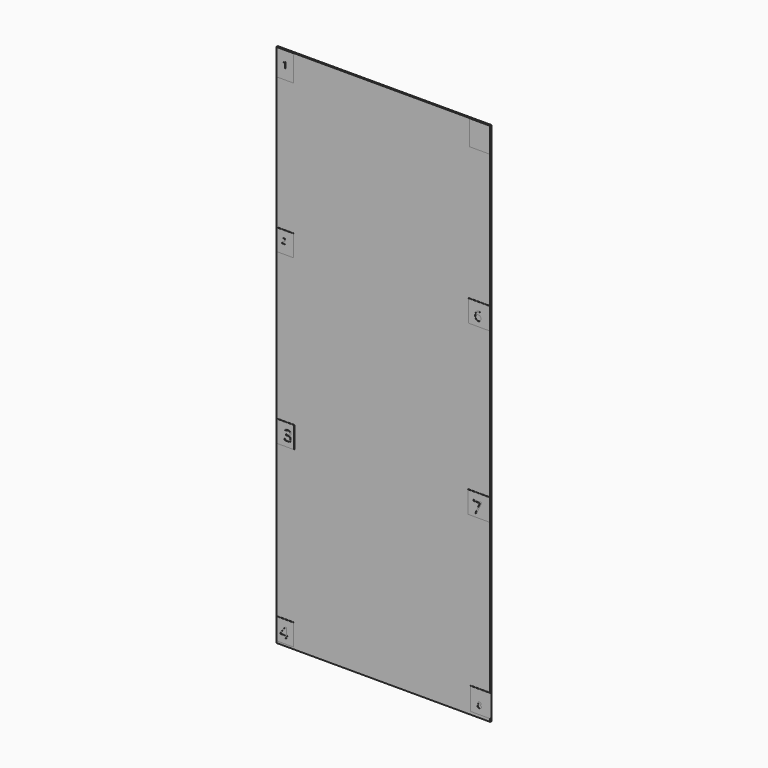
from build123d import *

# Parameters (mm, degrees)
F0_W         = 3500
F0_H         = 8600
F1_DEPTH     = 25
F2_W         = 335
F2_H         = 410
F2_W_2       = 360
F2_H_2       = 360
F2_W_3       = 345
F2_H_3       = 370
F2_W_4       = 350
F2_W_5       = 280
F2_H_4       = 430
F2_W_6       = 290
F2_H_5       = 355
F2_H_6       = 350
F2_TEXT_SIZE = 244.8439598083
F3_DEPTH     = 5


# Not quite as in the source:
# - Text() gives the source's letters only with a copy of the font that has no kerning and outlines rounded to 1/6400 em; it was checked with that copy


with BuildPart() as f1:
    # F0 (on Front) → F1 (new body)
    with BuildSketch(Plane.XZ):
        with Locations((-20.3130850568, 3129.9097295289)):
            Rectangle(F0_W, F0_H)
    extrude(amount=F1_DEPTH)

    # F2 (on face) → F3 (join)
    with BuildSketch(Plane.XZ.offset(25)):
        with Locations((1562.1869149432, 7224.9097295289)):
            Rectangle(F2_W, F2_H)
        with BuildLine():
            add(Edge.make_bspline(
                [(1530.7536032051, 7194.8450300843), (1544.4878190756, 7197.5995246321), (1558.1455212086, 7197.5995246321)],
                knots=[0, 0, 0, 1, 1, 1], degree=2))
            add(Edge.make_bspline(
                [(1558.1455212086, 7197.5995246321), (1585.7669804245, 7197.5995246321), (1601.6053240746, 7183.9035656303)],
                knots=[0, 0, 0, 1, 1, 1], degree=2))
            add(Edge.make_bspline(
                [(1601.6053240746, 7183.9035656303), (1617.4436677247, 7170.2076066285), (1617.4436677247, 7146.4118342847)],
                knots=[0, 0, 0, 1, 1, 1], degree=2))
            add(Edge.make_bspline(
                [(1617.4436677247, 7146.4118342847), (1617.4436677247, 7119.2877143621), (1600.1706914976, 7103.8510678336)],
                knots=[0, 0, 0, 1, 1, 1], degree=2))
            add(Edge.make_bspline(
                [(1600.1706914976, 7103.8510678336), (1582.8977152705, 7088.4144213051), (1552.5217615068, 7088.4144213051)],
                knots=[0, 0, 0, 1, 1, 1], degree=2))
            add(Edge.make_bspline(
                [(1552.5217615068, 7088.4144213051), (1522.9874588549, 7088.4144213051), (1507.4551701546, 7097.8638678789)],
                knots=[0, 0, 0, 1, 1, 1], degree=2))
            Line((1507.4551701546, 7097.8638678789), (1507.4551701546, 7116.9923022389))
            add(Edge.make_bspline(
                [(1507.4551701546, 7116.9923022389), (1515.7951675355, 7111.6363406181), (1528.2286498696, 7108.5757911205)],
                knots=[0, 0, 0, 1, 1, 1], degree=2))
            add(Edge.make_bspline(
                [(1528.2286498696, 7108.5757911205), (1540.6621322036, 7105.5152416229), (1552.7513027191, 7105.5152416229)],
                knots=[0, 0, 0, 1, 1, 1], degree=2))
            add(Edge.make_bspline(
                [(1552.7513027191, 7105.5152416229), (1573.7925805151, 7105.5152416229), (1585.4417970404, 7115.4428990558)],
                knots=[0, 0, 0, 1, 1, 1], degree=2))
            add(Edge.make_bspline(
                [(1585.4417970404, 7115.4428990558), (1597.0910135657, 7125.3705564886), (1597.0910135657, 7144.1546790302)],
                knots=[0, 0, 0, 1, 1, 1], degree=2))
            add(Edge.make_bspline(
                [(1597.0910135657, 7144.1546790302), (1597.0910135657, 7180.7282455266), (1552.2922202945, 7180.7282455266)],
                knots=[0, 0, 0, 1, 1, 1], degree=2))
            add(Edge.make_bspline(
                [(1552.2922202945, 7180.7282455266), (1540.9299302846, 7180.7282455266), (1521.9162665308, 7177.246870473)],
                knots=[0, 0, 0, 1, 1, 1], degree=2))
            Line((1521.9162665308, 7177.246870473), (1511.6251688451, 7183.8270518929))
            Line((1511.6251688451, 7183.8270518929), (1518.2053502649, 7265.6202372164))
            Line((1518.2053502649, 7265.6202372164), (1605.1249559969, 7265.6202372164))
            Line((1605.1249559969, 7265.6202372164), (1605.1249559969, 7247.3334539682))
            Line((1605.1249559969, 7247.3334539682), (1535.1913999766, 7247.3334539682))
            Line((1535.1913999766, 7247.3334539682), (1530.7536032051, 7194.8450300843))
        make_face(mode=Mode.SUBTRACT)
        with Locations((1549.6869149432, 1889.9097295289)):
            Rectangle(F2_W_2, F2_H_2)
        Polygon((1511.2107449418, 1764.8577690125), (1487.6480011735, 1764.8577690125), (1565.2206515272, 1932.5015685883), (1463.1837263393, 1932.5015685883), (1463.1837263393, 1952.0893799296), (1587.7589281752, 1952.0893799296), (1587.7589281752, 1935.0422470468), align=None, mode=Mode.SUBTRACT)
        with Locations((1581.1869149432, -935.0902704711)):
            Rectangle(F2_W_3, F2_H_3)
        with BuildLine():
            add(Edge.make_bspline(
                [(1538.5825815283, -940.5508573964), (1546.0325272592, -934.5624814002), (1558.5370683225, -934.5624814002)],
                knots=[0, 0, 0, 1, 1, 1], degree=2))
            add(Edge.make_bspline(
                [(1558.5370683225, -934.5624814002), (1571.2243056026, -934.5624814002), (1578.643801964, -940.459509288)],
                knots=[0, 0, 0, 1, 1, 1], degree=2))
            add(Edge.make_bspline(
                [(1578.643801964, -940.459509288), (1586.0632983254, -946.3565371758), (1586.0632983254, -956.7499219557)],
                knots=[0, 0, 0, 1, 1, 1], degree=2))
            add(Edge.make_bspline(
                [(1586.0632983254, -956.7499219557), (1586.0632983254, -963.6111798768), (1581.8206861789, -969.254463019)],
                knots=[0, 0, 0, 1, 1, 1], degree=2))
            add(Edge.make_bspline(
                [(1581.8206861789, -969.254463019), (1577.5780740325, -974.8977461612), (1568.2402673943, -979.526050321)],
                knots=[0, 0, 0, 1, 1, 1], degree=2))
            add(Edge.make_bspline(
                [(1568.2402673943, -979.526050321), (1579.5268336787, -984.9257385074), (1584.2870851062, -990.8532157647)],
                knots=[0, 0, 0, 1, 1, 1], degree=2))
            add(Edge.make_bspline(
                [(1584.2870851062, -990.8532157647), (1589.0473365337, -996.780693022), (1589.0473365337, -1004.5960311865)],
                knots=[0, 0, 0, 1, 1, 1], degree=2))
            add(Edge.make_bspline(
                [(1589.0473365337, -1004.5960311865), (1589.0473365337, -1016.1261924267), (1580.9884034134, -1023.0178997173)],
                knots=[0, 0, 0, 1, 1, 1], degree=2))
            add(Edge.make_bspline(
                [(1580.9884034134, -1023.0178997173), (1572.929470293, -1029.9096070078), (1558.9227603358, -1029.9096070078)],
                knots=[0, 0, 0, 1, 1, 1], degree=2))
            add(Edge.make_bspline(
                [(1558.9227603358, -1029.9096070078), (1544.0837676129, -1029.9096070078), (1536.0857332315, -1023.4035917306)],
                knots=[0, 0, 0, 1, 1, 1], degree=2))
            add(Edge.make_bspline(
                [(1536.0857332315, -1023.4035917306), (1528.0876988501, -1016.8975764533), (1528.0876988501, -1004.9614236202)],
                knots=[0, 0, 0, 1, 1, 1], degree=2))
            add(Edge.make_bspline(
                [(1528.0876988501, -1004.9614236202), (1528.0876988501, -989.046553176), (1547.4940969938, -980.1553372901)],
                knots=[0, 0, 0, 1, 1, 1], degree=2))
            add(Edge.make_bspline(
                [(1547.4940969938, -980.1553372901), (1538.7449781655, -975.2225394356), (1534.9388069814, -969.4777583951)],
                knots=[0, 0, 0, 1, 1, 1], degree=2))
            add(Edge.make_bspline(
                [(1534.9388069814, -969.4777583951), (1531.1326357974, -963.7329773547), (1531.1326357974, -956.6281244778)],
                knots=[0, 0, 0, 1, 1, 1], degree=2))
            add(Edge.make_bspline(
                [(1531.1326357974, -956.6281244778), (1531.1326357974, -946.5392333927), (1538.5825815283, -940.5508573964)],
                knots=[0, 0, 0, 1, 1, 1], degree=2))
        make_face(mode=Mode.SUBTRACT)
        with Locations((1554.6869149432, 4649.9097295289)):
            Rectangle(F2_W_4, F2_H_2)
        with BuildLine():
            add(Edge.make_bspline(
                [(1501.2481256078, 4567.1893796987), (1488.1472264727, 4583.9951059057), (1488.1472264727, 4613.9490269125)],
                knots=[0, 0, 0, 1, 1, 1], degree=2))
            add(Edge.make_bspline(
                [(1488.1472264727, 4613.9490269125), (1488.1472264727, 4656.4205338558), (1504.6534134696, 4677.4513394468)],
                knots=[0, 0, 0, 1, 1, 1], degree=2))
            add(Edge.make_bspline(
                [(1504.6534134696, 4677.4513394468), (1521.1596004665, 4698.4821450379), (1553.4783047107, 4698.4821450379)],
                knots=[0, 0, 0, 1, 1, 1], degree=2))
            add(Edge.make_bspline(
                [(1553.4783047107, 4698.4821450379), (1564.6085511479, 4698.4821450379), (1571.0092311104, 4696.6218488912)],
                knots=[0, 0, 0, 1, 1, 1], degree=2))
            Line((1571.0092311104, 4696.6218488912), (1571.0092311104, 4682.5277407964))
            add(Edge.make_bspline(
                [(1571.0092311104, 4682.5277407964), (1563.4103943076, 4684.9871153633), (1553.6674873696, 4684.9871153633)],
                knots=[0, 0, 0, 1, 1, 1], degree=2))
            add(Edge.make_bspline(
                [(1553.6674873696, 4684.9871153633), (1530.4926116433, 4684.9871153633), (1518.2745649169, 4670.5619376153)],
                knots=[0, 0, 0, 1, 1, 1], degree=2))
            add(Edge.make_bspline(
                [(1518.2745649169, 4670.5619376153), (1506.0565181904, 4656.1367598673), (1504.8898917933, 4625.1738646792)],
                knots=[0, 0, 0, 1, 1, 1], degree=2))
            Line((1504.8898917933, 4625.1738646792), (1506.0565181904, 4625.1738646792))
            add(Edge.make_bspline(
                [(1506.0565181904, 4625.1738646792), (1516.9029906392, 4642.137243102), (1540.361640354, 4642.137243102)],
                knots=[0, 0, 0, 1, 1, 1], degree=2))
            add(Edge.make_bspline(
                [(1540.361640354, 4642.137243102), (1559.7843933437, 4642.137243102), (1570.9619354457, 4630.4079182446)],
                knots=[0, 0, 0, 1, 1, 1], degree=2))
            add(Edge.make_bspline(
                [(1570.9619354457, 4630.4079182446), (1582.1394775477, 4618.6785933872), (1582.1394775477, 4598.5937010911)],
                knots=[0, 0, 0, 1, 1, 1], degree=2))
            add(Edge.make_bspline(
                [(1582.1394775477, 4598.5937010911), (1582.1394775477, 4576.1124951144), (1569.8741351565, 4563.2480743031)],
                knots=[0, 0, 0, 1, 1, 1], degree=2))
            add(Edge.make_bspline(
                [(1569.8741351565, 4563.2480743031), (1557.6087927653, 4550.3836534917), (1536.7041089469, 4550.3836534917)],
                knots=[0, 0, 0, 1, 1, 1], degree=2))
            add(Edge.make_bspline(
                [(1536.7041089469, 4550.3836534917), (1514.3490247428, 4550.3836534917), (1501.2481256078, 4567.1893796987)],
                knots=[0, 0, 0, 1, 1, 1], degree=2))
        make_face(mode=Mode.SUBTRACT)
        with Locations((-1630.3130850568, 7214.9097295289)):
            Rectangle(F2_W_5, F2_H_4)
        with BuildLine():
            Line((-1613.7520122445, 7270.6857842083), (-1613.7520122445, 7168.0779457092))
            Line((-1613.7520122445, 7168.0779457092), (-1625.1154541969, 7168.0779457092))
            Line((-1625.1154541969, 7168.0779457092), (-1625.1154541969, 7241.1992243595))
            add(Edge.make_bspline(
                [(-1625.1154541969, 7241.1992243595), (-1625.1154541969, 7250.3393841907), (-1624.5540193179, 7258.4689612397)],
                knots=[0, 0, 0, 1, 1, 1], degree=2))
            add(Edge.make_bspline(
                [(-1624.5540193179, 7258.4689612397), (-1626.0137500034, 7256.9867731589), (-1627.8440277092, 7255.3810694048)],
                knots=[0, 0, 0, 1, 1, 1], degree=2))
            add(Edge.make_bspline(
                [(-1627.8440277092, 7255.3810694048), (-1629.674305415, 7253.7753656507), (-1644.5411010128, 7241.693287053)],
                knots=[0, 0, 0, 1, 1, 1], degree=2))
            Line((-1644.5411010128, 7241.693287053), (-1650.7168846826, 7249.688119731))
            Line((-1650.7168846826, 7249.688119731), (-1623.5658939307, 7270.6857842083))
            Line((-1623.5658939307, 7270.6857842083), (-1613.7520122445, 7270.6857842083))
        make_face(mode=Mode.SUBTRACT)
        with Locations((-1625.3130850568, 1892.4097295289)):
            Rectangle(F2_W_6, F2_H_5)
        with BuildLine():
            add(Edge.make_bspline(
                [(-1540.9848357861, 1964.2068696622), (-1527.0048653086, 1952.6705525609), (-1527.0048653086, 1932.5530340688)],
                knots=[0, 0, 0, 1, 1, 1], degree=2))
            add(Edge.make_bspline(
                [(-1527.0048653086, 1932.5530340688), (-1527.0048653086, 1915.9589227703), (-1536.3059025775, 1905.4265872886)],
                knots=[0, 0, 0, 1, 1, 1], degree=2))
            add(Edge.make_bspline(
                [(-1536.3059025775, 1905.4265872886), (-1545.6069398464, 1894.8942518069), (-1562.6556843312, 1891.3329585145)],
                knots=[0, 0, 0, 1, 1, 1], degree=2))
            Line((-1562.6556843312, 1891.3329585145), (-1562.6556843312, 1890.3858060431))
            add(Edge.make_bspline(
                [(-1562.6556843312, 1890.3858060431), (-1541.8183299609, 1887.809551321), (-1531.7595707149, 1877.1446144933)],
                knots=[0, 0, 0, 1, 1, 1], degree=2))
            add(Edge.make_bspline(
                [(-1531.7595707149, 1877.1446144933), (-1521.7008114689, 1866.4796776656), (-1521.7008114689, 1849.2036165877)],
                knots=[0, 0, 0, 1, 1, 1], degree=2))
            add(Edge.make_bspline(
                [(-1521.7008114689, 1849.2036165877), (-1521.7008114689, 1824.4639940353), (-1538.8632142502, 1811.1280872383)],
                knots=[0, 0, 0, 1, 1, 1], degree=2))
            add(Edge.make_bspline(
                [(-1538.8632142502, 1811.1280872383), (-1556.0256170316, 1797.7921804413), (-1587.6226234767, 1797.7921804413)],
                knots=[0, 0, 0, 1, 1, 1], degree=2))
            add(Edge.make_bspline(
                [(-1587.6226234767, 1797.7921804413), (-1601.3752773611, 1797.7921804413), (-1612.7979361659, 1799.8759158783)],
                knots=[0, 0, 0, 1, 1, 1], degree=2))
            add(Edge.make_bspline(
                [(-1612.7979361659, 1799.8759158783), (-1624.2205949707, 1801.9596513154), (-1634.9802470456, 1807.1500468585)],
                knots=[0, 0, 0, 1, 1, 1], degree=2))
            Line((-1634.9802470456, 1807.1500468585), (-1634.9802470456, 1825.8657796929))
            add(Edge.make_bspline(
                [(-1634.9802470456, 1825.8657796929), (-1623.7280756856, 1820.2965231612), (-1610.9983464703, 1817.3982365988)],
                knots=[0, 0, 0, 1, 1, 1], degree=2))
            add(Edge.make_bspline(
                [(-1610.9983464703, 1817.3982365988), (-1598.268617255, 1814.4999500364), (-1586.9027875985, 1814.4999500364)],
                knots=[0, 0, 0, 1, 1, 1], degree=2))
            add(Edge.make_bspline(
                [(-1586.9027875985, 1814.4999500364), (-1542.0456465541, 1814.4999500364), (-1542.0456465541, 1849.6582497739)],
                knots=[0, 0, 0, 1, 1, 1], degree=2))
            add(Edge.make_bspline(
                [(-1542.0456465541, 1849.6582497739), (-1542.0456465541, 1881.1794840213), (-1591.5248916588, 1881.1794840213)],
                knots=[0, 0, 0, 1, 1, 1], degree=2))
            Line((-1591.5248916588, 1881.1794840213), (-1608.5736361436, 1881.1794840213))
            Line((-1608.5736361436, 1881.1794840213), (-1608.5736361436, 1898.0766841107))
            Line((-1608.5736361436, 1898.0766841107), (-1591.2975750657, 1898.0766841107))
            add(Edge.make_bspline(
                [(-1591.2975750657, 1898.0766841107), (-1571.0663982771, 1898.0766841107), (-1559.2269923848, 1907.0178034405)],
                knots=[0, 0, 0, 1, 1, 1], degree=2))
            add(Edge.make_bspline(
                [(-1559.2269923848, 1907.0178034405), (-1547.3875864926, 1915.9589227703), (-1547.3875864926, 1931.8331981906)],
                knots=[0, 0, 0, 1, 1, 1], degree=2))
            add(Edge.make_bspline(
                [(-1547.3875864926, 1931.8331981906), (-1547.3875864926, 1944.4871552082), (-1556.0824461799, 1951.7234000895)],
                knots=[0, 0, 0, 1, 1, 1], degree=2))
            add(Edge.make_bspline(
                [(-1556.0824461799, 1951.7234000895), (-1564.7773058671, 1958.9596449708), (-1579.704428816, 1958.9596449708)],
                knots=[0, 0, 0, 1, 1, 1], degree=2))
            add(Edge.make_bspline(
                [(-1579.704428816, 1958.9596449708), (-1591.0702584725, 1958.9596449708), (-1601.1290177186, 1955.8719279141)],
                knots=[0, 0, 0, 1, 1, 1], degree=2))
            add(Edge.make_bspline(
                [(-1601.1290177186, 1955.8719279141), (-1611.1877769646, 1952.7842108574), (-1624.1069366742, 1944.4871552082)],
                knots=[0, 0, 0, 1, 1, 1], degree=2))
            Line((-1624.1069366742, 1944.4871552082), (-1634.0330945742, 1957.7472898074))
            add(Edge.make_bspline(
                [(-1634.0330945742, 1957.7472898074), (-1623.3871007959, 1966.1580037533), (-1609.4829025161, 1970.9505952584)],
                knots=[0, 0, 0, 1, 1, 1], degree=2))
            add(Edge.make_bspline(
                [(-1609.4829025161, 1970.9505952584), (-1595.5787042363, 1975.7431867636), (-1580.1590620023, 1975.7431867636)],
                knots=[0, 0, 0, 1, 1, 1], degree=2))
            add(Edge.make_bspline(
                [(-1580.1590620023, 1975.7431867636), (-1554.9648062636, 1975.7431867636), (-1540.9848357861, 1964.2068696622)],
                knots=[0, 0, 0, 1, 1, 1], degree=2))
        make_face(mode=Mode.SUBTRACT)
        with Locations((-1630.3130850568, -957.5902704711)):
            Rectangle(F2_W_5, F2_H_5)
        Polygon((-1583.7438841894, -996.8644978427), (-1583.7438841894, -1013.144360312), (-1607.1289408719, -1013.144360312), (-1607.1289408719, -1049.3601560593), (-1624.2710841923, -1049.3601560593), (-1624.2710841923, -1013.144360312), (-1700.9106062404, -1013.144360312), (-1700.9106062404, -997.5198312895), (-1626.0991195967, -890.9074268563), (-1607.1289408719, -890.9074268563), (-1607.1289408719, -996.8644978427), align=None, mode=Mode.SUBTRACT)
        with Locations((-1630.3130850568, 4654.9097295289)):
            Rectangle(F2_W_5, F2_H_6)
        with BuildLine():
            Line((-1617.2033854657, 4636.0510933316), (-1617.2033854657, 4626.6403198242))
            Line((-1617.2033854657, 4626.6403198242), (-1675.9571335796, 4626.6403198242))
            Line((-1675.9571335796, 4626.6403198242), (-1675.9571335796, 4635.3858827303))
            Line((-1675.9571335796, 4635.3858827303), (-1652.4204173022, 4659.0399891138))
            add(Edge.make_bspline(
                [(-1652.4204173022, 4659.0399891138), (-1641.6596575744, 4669.9377039654), (-1638.2357794791, 4674.5843956661)],
                knots=[0, 0, 0, 1, 1, 1], degree=2))
            add(Edge.make_bspline(
                [(-1638.2357794791, 4674.5843956661), (-1634.8119013839, 4679.2310873667), (-1633.0999623363, 4683.6332163463)],
                knots=[0, 0, 0, 1, 1, 1], degree=2))
            add(Edge.make_bspline(
                [(-1633.0999623363, 4683.6332163463), (-1631.3880232887, 4688.0353453259), (-1631.3880232887, 4693.1026849068)],
                knots=[0, 0, 0, 1, 1, 1], degree=2))
            add(Edge.make_bspline(
                [(-1631.3880232887, 4693.1026849068), (-1631.3880232887, 4700.2634813802), (-1635.7314572152, 4704.4503951652)],
                knots=[0, 0, 0, 1, 1, 1], degree=2))
            add(Edge.make_bspline(
                [(-1635.7314572152, 4704.4503951652), (-1640.0748911417, 4708.6373089502), (-1647.7835081104, 4708.6373089502)],
                knots=[0, 0, 0, 1, 1, 1], degree=2))
            add(Edge.make_bspline(
                [(-1647.7835081104, 4708.6373089502), (-1653.3399731335, 4708.6373089502), (-1658.3290526436, 4706.7981972877)],
                knots=[0, 0, 0, 1, 1, 1], degree=2))
            add(Edge.make_bspline(
                [(-1658.3290526436, 4706.7981972877), (-1663.3181321538, 4704.9590856251), (-1669.4224176721, 4700.1265262564)],
                knots=[0, 0, 0, 1, 1, 1], degree=2))
            Line((-1669.4224176721, 4700.1265262564), (-1674.8027975361, 4707.0329774999))
            add(Edge.make_bspline(
                [(-1674.8027975361, 4707.0329774999), (-1662.4572713756, 4717.3046117855), (-1647.9008982165, 4717.3046117855)],
                knots=[0, 0, 0, 1, 1, 1], degree=2))
            add(Edge.make_bspline(
                [(-1647.9008982165, 4717.3046117855), (-1635.3010268261, 4717.3046117855), (-1628.1500128615, 4710.8579384577)],
                knots=[0, 0, 0, 1, 1, 1], degree=2))
            add(Edge.make_bspline(
                [(-1628.1500128615, 4710.8579384577), (-1620.9989988969, 4704.4112651298), (-1620.9989988969, 4693.5331152959)],
                knots=[0, 0, 0, 1, 1, 1], degree=2))
            add(Edge.make_bspline(
                [(-1620.9989988969, 4693.5331152959), (-1620.9989988969, 4685.0223326021), (-1625.7728632126, 4676.7072000851)],
                knots=[0, 0, 0, 1, 1, 1], degree=2))
            add(Edge.make_bspline(
                [(-1625.7728632126, 4676.7072000851), (-1630.5467275282, 4668.3920675682), (-1643.6161593431, 4655.6748060717)],
                knots=[0, 0, 0, 1, 1, 1], degree=2))
            Line((-1643.6161593431, 4655.6748060717), (-1663.18117703, 4636.5402187738))
            Line((-1663.18117703, 4636.5402187738), (-1663.18117703, 4636.0510933316))
            Line((-1663.18117703, 4636.0510933316), (-1617.2033854657, 4636.0510933316))
        make_face(mode=Mode.SUBTRACT)
        with Locations((1491.540312767, 7090.8246040344)):
            Text('5', F2_TEXT_SIZE, font='Open Sans', text_align=(TextAlign.LEFT, TextAlign.BOTTOM))
    extrude(amount=F3_DEPTH)


solid = f1.part
